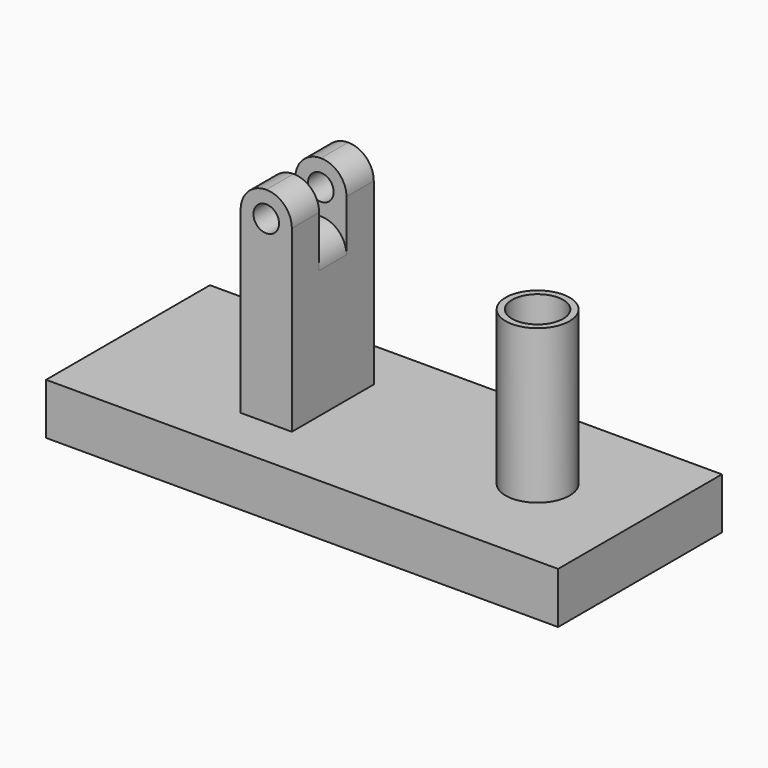
from build123d import *

# Parameters (mm, degrees)
F0_W     = 127
F0_H     = 50.8
F1_DEPTH = 12.7
F2_R     = 7.9375
F2_R_2   = 6.35
F2_W     = 12.7
F2_H     = 25.4
F3_DEPTH = 38.1
F4_W     = 12.7
F4_H     = 8.466582
F4_H_2   = 8.46582
F5_DEPTH = 12.7
F6_R     = 6.34999
F7_R     = 3.175
F8_DEPTH = 25.4


# Not quite as in the source:
# - a fillet or chamfer is up to 0.001 mm smaller than in the source, because OpenCascade refuses the exact size


with BuildPart() as f1:
    # F0 (on Top) → F1 (new body)
    with BuildSketch(Plane.XY):
        with Locations((-63.5, 25.4)):
            Rectangle(F0_W, F0_H)
    extrude(amount=F1_DEPTH)

    # F2 (on face) → F3 (join)
    with BuildSketch(Plane.XY.offset(12.7)):
        with Locations((-25.4, 25.4)):
            Circle(F2_R)
        with Locations((-25.4, 25.4)):
            Circle(F2_R_2, mode=Mode.SUBTRACT)
        with Locations((-82.55, 25.4)):
            Rectangle(F2_W, F2_H)
    extrude(amount=F3_DEPTH)

    # F4 (on face) → F5 (join)
    with BuildSketch(Plane.XY.offset(50.8)):
        with Locations((-82.55, 33.866709)):
            Rectangle(F4_W, F4_H)
        with Locations((-82.55, 16.93291)):
            Rectangle(F4_W, F4_H_2)
    extrude(amount=F5_DEPTH)

    # F6 (radius 6.35 in the source; OpenCascade refuses exactly that, so slightly less here)
    f6_edges = [f1.edges().sort_by_distance(p)[0] for p in [
        (-88.9, 33.866709, 63.5),
        (-88.9, 16.93291, 63.5),
        (-76.2, 33.866709, 63.5),
        (-76.2, 16.93291, 63.5),
        (-88.9, 25.399619, 50.8),
        (-76.2, 25.399619, 50.8),
    ]]
    fillet(f6_edges, radius=F6_R)

    # F7 (on face) → F8 (cut)
    with BuildSketch(Plane(origin=(0, 38.1, 0), x_dir=(-1, 0, 0), z_dir=(0, 1, 0))):
        with Locations((82.55, 57.15)):
            Circle(F7_R)
    extrude(amount=-F8_DEPTH, mode=Mode.SUBTRACT)


solid = f1.part
